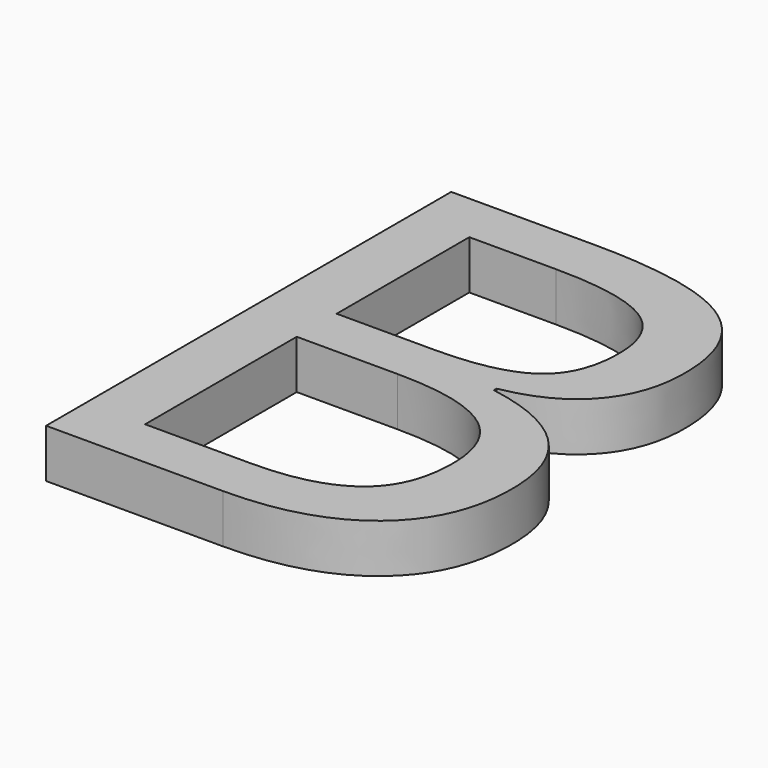
from build123d import *

# Parameters (mm, degrees)
F0_TEXT_SIZE = 11.0995656777
F1_DEPTH     = 0.762


# Not quite as in the source:
# - Text() gives the source's letters only with a copy of the font that has no kerning and outlines rounded to 1/6400 em; it was checked with that copy


with BuildPart() as f1:
    # F0 (on Top) → F1 (new body)
    with BuildSketch(Plane.XY):
        with Locations((-7.2996987402, 0)):
            Text('B', F0_TEXT_SIZE, font='Open Sans', text_align=(TextAlign.LEFT, TextAlign.BOTTOM))
    extrude(amount=F1_DEPTH)


solid = f1.part
